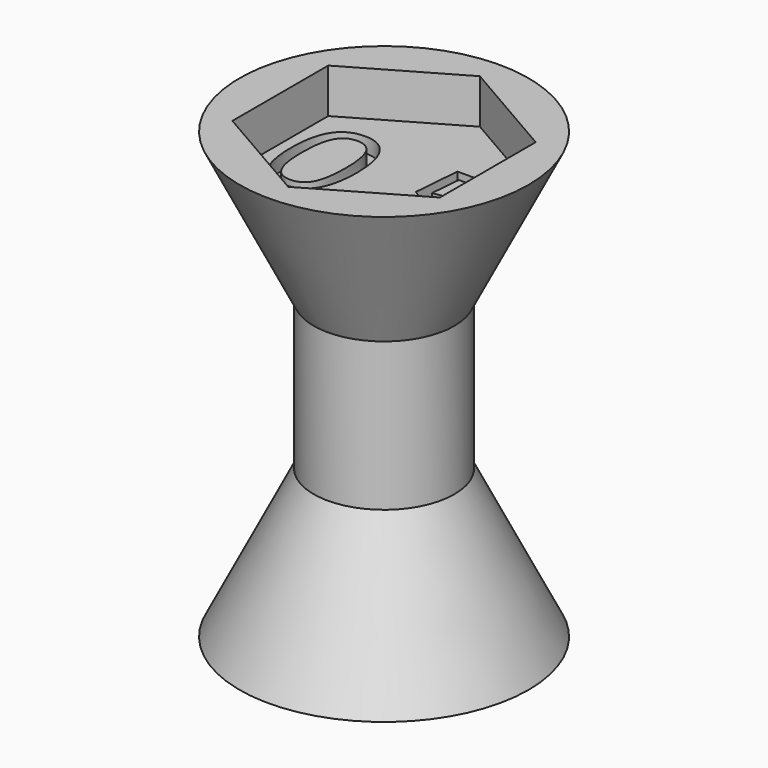
from build123d import *

# Parameters (mm, degrees)
F3_DEPTH     = 3
F4_TEXT_SIZE = 9.5280105867
F5_DEPTH     = 1


# Not quite as in the source:
# - Text() gives the source's letters only with a copy of the font that has no kerning and outlines rounded to 1/6400 em; it was checked with that copy


with BuildPart() as f1:
    # F0 (on Front) → F1 (revolve)
    with BuildSketch(Plane.XZ):
        Polygon((9.75, 15), (0, 15), (0, -15), (9.75, -15), (4.75, -5), (4.75, 5), align=None)
    revolve(axis=Axis((0, 0, 0), (0, 0, -1)))

    # F2 (on face) → F3 (cut)
    with BuildSketch(Plane.XY.offset(15)):
        Polygon((7, 4.0414518843), (0, 8.0829037687), (-7, 4.0414518843), (-7, -4.0414518843), (0, -8.0829037687), (7, -4.0414518843), align=None)
    extrude(amount=-F3_DEPTH, mode=Mode.SUBTRACT)

    # F4 (on face) → F5 (cut)
    with BuildSketch(Plane.XY.offset(12)):
        with Locations((-6.75, -3.4519142963)):
            Text('0.5', F4_TEXT_SIZE, font='Open Sans', text_align=(TextAlign.LEFT, TextAlign.BOTTOM))
    extrude(amount=-F5_DEPTH, mode=Mode.SUBTRACT)


solid = f1.part
